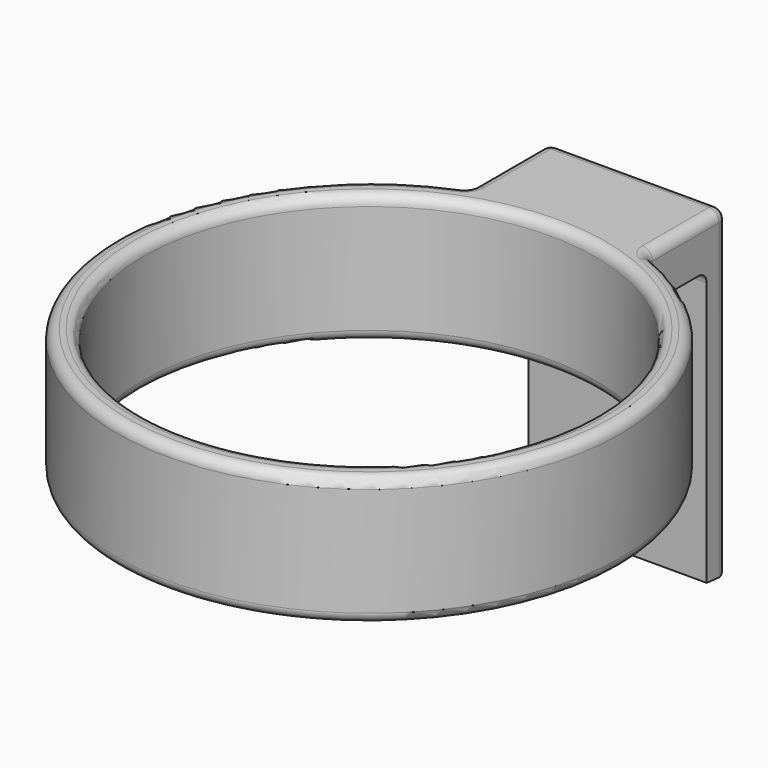
from build123d import *

# Parameters (mm, degrees)
F0_R     = 49.53
F0_R_2   = 44.45
F1_DEPTH = 25.4
F3_DEPTH = 17.5
F4_R     = 2


with BuildPart() as f1:
    # F0 (on Top) → F1 (new body)
    with BuildSketch(Plane.XY):
        Circle(F0_R)
        Circle(F0_R_2, mode=Mode.SUBTRACT)
    extrude(amount=F1_DEPTH)

    # F2 (on Right) → F3 (join, symmetric)
    with BuildSketch(Plane.YZ):
        Polygon((66.002712847, 25.4), (45.682712847, 25.4), (45.682712847, 16.2404105067), (60.96, 16.2404105067), (60.96, -37.6108922064), (66.002712847, -38.1), align=None)
    extrude(amount=F3_DEPTH, both=True)

    # F4
    f4_edges = [f1.edges().sort_by_distance(p)[0] for p in [
        (0, 60.96, 16.240411),
        (0, 49.53, 16.240411),
        (17.5, 46.335417, 20.820205),
        (-17.5, 46.335417, 20.820205),
        (0, 66.002713, 25.4),
        (-44.45, 0, 25.4),
        (-49.53, 0, 0),
        (49.53, 0, 12.7),
        (-28.164214, -40.743072, 25.4),
        (40.743072, 28.164214, 25.4),
        (44.45, 0, 12.7),
        (-44.45, 0, 0),
        (-17.5, 66.002713, -6.35),
        (17.5, 66.002713, -6.35),
        (0, 66.002713, -38.1),
        (17.5, 56.169065, 25.4),
        (-17.5, 56.169065, 25.4),
    ]]
    fillet(f4_edges, radius=F4_R)


solid = f1.part
